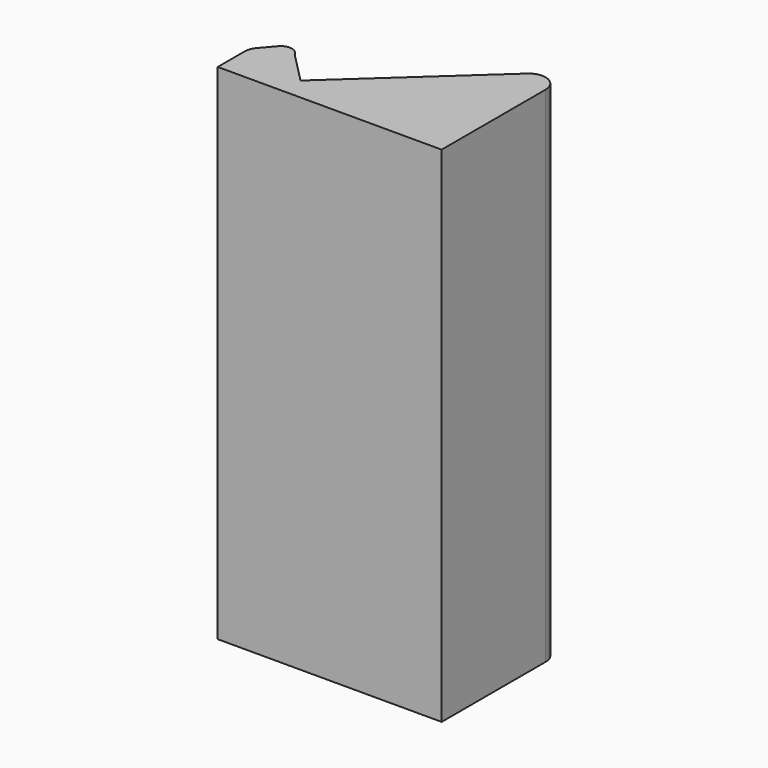
from build123d import *

# Parameters (mm, degrees)
F1_DEPTH    = 90
F2_R        = 3
F3_T1_DEPTH = 113.3705433716


# Not quite as in the source:
# - a fillet or chamfer that OpenCascade refuses, or shapes differently, is made with other operations: its cross-section is extruded or revolved along the edge and cut away or added


with BuildPart() as f1:
    # F0 (on Top) → F1 (new body)
    with BuildSketch(Plane.XY):
        Polygon((-20, -17.5), (20, -17.5), (20, 12.5313148581), (-8.4129939735, -13.5), (-14.0197880107, -7.7935246759), (-14.2998851884, -3.8033435308), (-20, -10.4466760531), align=None)
    extrude(amount=F1_DEPTH)

    # F2
    f2_edges = [f1.edges().sort_by_distance(p)[0] for p in [
        (-20, -10.446676, 45),
        (20, 12.531315, 45),
    ]]
    fillet(f2_edges, radius=F2_R)

    # F3: fillet of radius 2 on 1 edges, made by hand

    # F3_s2 → F3_t1 (cut)
    with BuildSketch(Plane.XY.offset(-11.6852716858)):
        with BuildLine():
            ThreePointArc((-17.3435489028, -7.3506528059), (-15.5615402204, -6.6705242909), (-14.0197880107, -7.7935246759))
            Line((-14.0197880107, -7.7935246759), (-14.2998851884, -3.8033435308))
            Line((-14.2998851884, -3.8033435308), (-17.3435489028, -7.3506528059))
        make_face()
    extrude(amount=F3_T1_DEPTH, mode=Mode.SUBTRACT)


solid = f1.part
